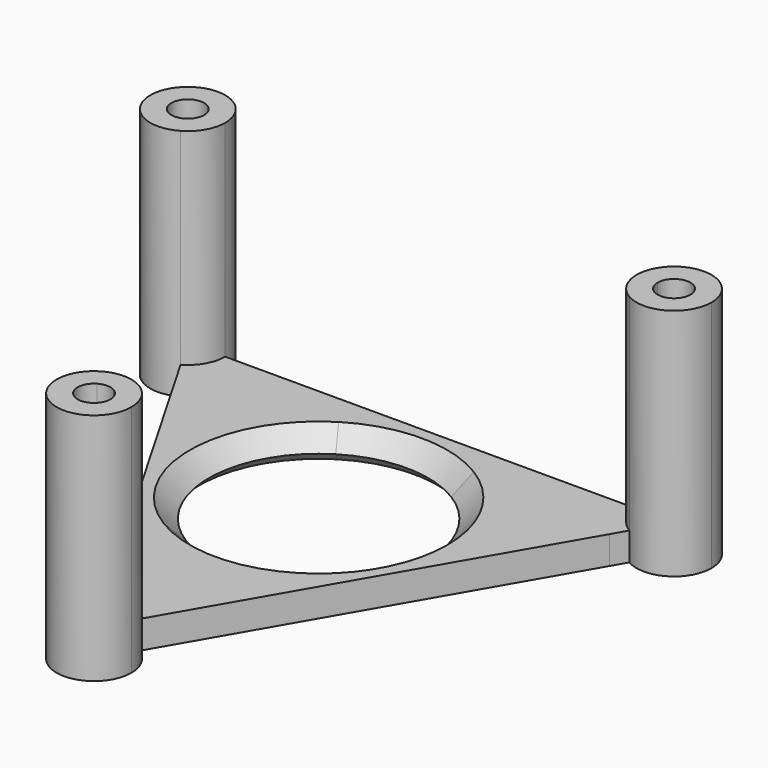
from build123d import *

# Parameters (mm, degrees)
F1_DEPTH = 3
F2_DEPTH = 25
F3_SIZE  = 1
F4_SIZE  = 1.99999


# Not quite as in the source:
# - a fillet or chamfer is up to 0.001 mm smaller than in the source, because OpenCascade refuses the exact size


with BuildPart() as f1:
    # F0 (on Top) → F1 (new body)
    with BuildSketch(Plane.XY):
        with BuildLine():
            ThreePointArc((-6.1694813396, 10), (0, 11.75), (6.1694813396, 10))
            Line((6.1694813396, 10), (23.0940107676, 10))
            Line((23.0940107676, 10), (23.9807621135, 11.5358983849))
            ThreePointArc((23.9807621135, 11.5358983849), (22.5166604984, 13), (21.9807621135, 15))
            Line((21.9807621135, 15), (-21.9807621135, 15))
            ThreePointArc((-21.9807621135, 15), (-22.5166604984, 13), (-23.9807621135, 11.5358983849))
            Line((-23.9807621135, 11.5358983849), (-23.0940107676, 10))
            Line((-23.0940107676, 10), (-6.1694813396, 10))
        make_face()
        with BuildLine():
            ThreePointArc((-6.1694813396, -10), (-11.75, 0), (-6.1694813396, 10))
            Line((-6.1694813396, 10), (-23.0940107676, 10))
            Line((-23.0940107676, 10), (-11.5470053838, -10))
            Line((-11.5470053838, -10), (-6.1694813396, -10))
        make_face()
        with BuildLine():
            Line((11.5470053838, -10), (6.1694813396, -10))
            ThreePointArc((6.1694813396, -10), (0, -11.75), (-6.1694813396, -10))
            Line((-6.1694813396, -10), (-11.5470053838, -10))
            Line((-11.5470053838, -10), (-2, -26.5358983849))
            ThreePointArc((-2, -26.5358983849), (0, -26), (2, -26.5358983849))
            Line((2, -26.5358983849), (11.5470053838, -10))
        make_face()
        with BuildLine():
            ThreePointArc((6.1694813396, 10), (10.2604557828, 5.725866496), (11.75, 0))
            ThreePointArc((11.75, 0), (10.2604557828, -5.725866496), (6.1694813396, -10))
            Line((6.1694813396, -10), (11.5470053838, -10))
            Line((11.5470053838, -10), (23.0940107676, 10))
            Line((23.0940107676, 10), (6.1694813396, 10))
        make_face()
    extrude(amount=F1_DEPTH)



with BuildPart() as f1b:
    # F0 (on Top) → F1, piece 2 (new body)
    with BuildSketch(Plane.XY):
        with BuildLine():
            ThreePointArc((1.75, -30), (1.5155444566, -29.125), (0.875, -28.4844555434))
            Line((0.875, -28.4844555434), (0, -30))
            Line((0, -30), (-0.875, -28.4844555434))
            ThreePointArc((-0.875, -28.4844555434), (-0.875, -31.5155444566), (1.75, -30))
        make_face()
        with BuildLine():
            Line((0, -30), (0.875, -28.4844555434))
            ThreePointArc((0.875, -28.4844555434), (0, -28.25), (-0.875, -28.4844555434))
            Line((-0.875, -28.4844555434), (0, -30))
        make_face()
    extrude(amount=F1_DEPTH)


with BuildPart() as f1c:
    # F0 (on Top) → F1, piece 3 (new body)
    with BuildSketch(Plane.XY):
        with BuildLine():
            ThreePointArc((24.2307621135, 15), (24.4652176569, 14.125), (25.1057621135, 13.4844555434))
            Line((25.1057621135, 13.4844555434), (25.9807621135, 15))
            Line((25.9807621135, 15), (24.2307621135, 15))
        make_face()
        with BuildLine():
            Line((25.9807621135, 15), (25.1057621135, 13.4844555434))
            ThreePointArc((25.1057621135, 13.4844555434), (26.8557621135, 13.4844555434), (27.7307621135, 15))
            ThreePointArc((27.7307621135, 15), (25.9807621135, 16.75), (24.2307621135, 15))
            Line((24.2307621135, 15), (25.9807621135, 15))
        make_face()
    extrude(amount=F1_DEPTH)


with BuildPart() as f1d:
    # F0 (on Top) → F1, piece 4 (new body)
    with BuildSketch(Plane.XY):
        with BuildLine():
            Line((-25.9807621135, 15), (-25.1057621135, 13.4844555434))
            ThreePointArc((-25.1057621135, 13.4844555434), (-24.4652176569, 14.125), (-24.2307621135, 15))
            Line((-24.2307621135, 15), (-25.9807621135, 15))
        make_face()
        with BuildLine():
            ThreePointArc((-24.2307621135, 15), (-27.4963065702, 15.875), (-25.1057621135, 13.4844555434))
            Line((-25.1057621135, 13.4844555434), (-25.9807621135, 15))
            Line((-25.9807621135, 15), (-24.2307621135, 15))
        make_face()
    extrude(amount=F1_DEPTH)


with BuildPart() as f1_1:
    add(f1.part)

    add(f1b.part)  # F2 merges F1b

    add(f1c.part)  # F2 merges F1c

    add(f1d.part)  # F2 merges F1d
    # F0 (on Top) → F2 (join)
    with BuildSketch(Plane.XY):
        with BuildLine():
            Line((-25.1057621135, 13.4844555434), (-23.9807621135, 11.5358983849))
            ThreePointArc((-23.9807621135, 11.5358983849), (-22.5166604984, 13), (-21.9807621135, 15))
            Line((-21.9807621135, 15), (-24.2307621135, 15))
            ThreePointArc((-24.2307621135, 15), (-24.4652176569, 14.125), (-25.1057621135, 13.4844555434))
        make_face()
        with BuildLine():
            ThreePointArc((-21.9807621135, 15), (-29.4448637287, 17), (-23.9807621135, 11.5358983849))
            Line((-23.9807621135, 11.5358983849), (-25.1057621135, 13.4844555434))
            ThreePointArc((-25.1057621135, 13.4844555434), (-27.4963065702, 15.875), (-24.2307621135, 15))
            Line((-24.2307621135, 15), (-21.9807621135, 15))
        make_face()
        with BuildLine():
            ThreePointArc((21.9807621135, 15), (22.5166604984, 13), (23.9807621135, 11.5358983849))
            Line((23.9807621135, 11.5358983849), (25.1057621135, 13.4844555434))
            ThreePointArc((25.1057621135, 13.4844555434), (24.4652176569, 14.125), (24.2307621135, 15))
            Line((24.2307621135, 15), (21.9807621135, 15))
        make_face()
        with BuildLine():
            Line((25.1057621135, 13.4844555434), (23.9807621135, 11.5358983849))
            ThreePointArc((23.9807621135, 11.5358983849), (27.9807621135, 11.5358983849), (29.9807621135, 15))
            ThreePointArc((29.9807621135, 15), (25.9807621135, 19), (21.9807621135, 15))
            Line((21.9807621135, 15), (24.2307621135, 15))
            ThreePointArc((24.2307621135, 15), (25.9807621135, 16.75), (27.7307621135, 15))
            ThreePointArc((27.7307621135, 15), (26.8557621135, 13.4844555434), (25.1057621135, 13.4844555434))
        make_face()
        with BuildLine():
            Line((0.875, -28.4844555434), (2, -26.5358983849))
            ThreePointArc((2, -26.5358983849), (0, -26), (-2, -26.5358983849))
            Line((-2, -26.5358983849), (-0.875, -28.4844555434))
            ThreePointArc((-0.875, -28.4844555434), (0, -28.25), (0.875, -28.4844555434))
        make_face()
        with BuildLine():
            ThreePointArc((4, -30), (3.4641016151, -28), (2, -26.5358983849))
            Line((2, -26.5358983849), (0.875, -28.4844555434))
            ThreePointArc((0.875, -28.4844555434), (1.5155444566, -29.125), (1.75, -30))
            ThreePointArc((1.75, -30), (-0.875, -31.5155444566), (-0.875, -28.4844555434))
            Line((-0.875, -28.4844555434), (-2, -26.5358983849))
            ThreePointArc((-2, -26.5358983849), (-2, -33.4641016151), (4, -30))
        make_face()
    extrude(amount=F2_DEPTH)

    # F3
    f3_edges = [f1_1.edges().sort_by_distance(p)[0] for p in [
        (-6.169481, -10, 0),
    ]]
    chamfer(f3_edges, length=F3_SIZE)

    # F4 (size 2 in the source; OpenCascade refuses exactly that, so slightly less here)
    f4_edges = [f1_1.edges().sort_by_distance(p)[0] for p in [
        (-6.169481, -10, 3),
    ]]
    chamfer(f4_edges, length=F4_SIZE)


solid = f1_1.part
